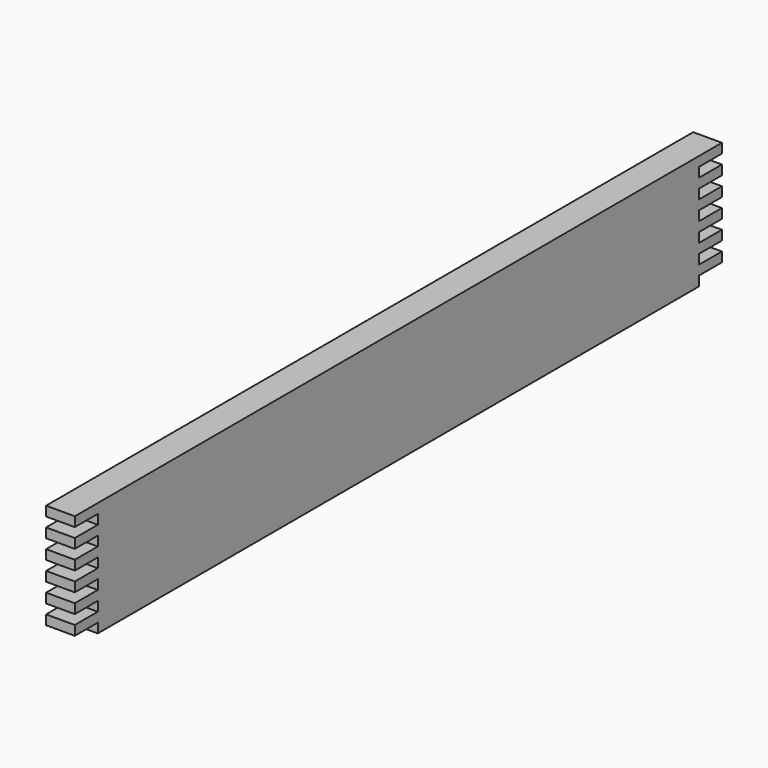
from build123d import *

# Parameters (mm, degrees)
F0_W     = 19.05
F0_H     = 76.2
F1_DEPTH = 268.351
F2_W     = 19.05
F2_H     = 6.35
F3_DEPTH = 19.051


# Not quite as in the source:
# - a pattern or mirror of a feature is missing from the dataset's text; its kind, count and spacing are read off the source's solid


with BuildPart() as f1:
    # F0 (on Front) → F1 (new body, symmetric)
    with BuildSketch(Plane.XZ):
        Rectangle(F0_W, F0_H)
    extrude(amount=F1_DEPTH, both=True)

    # F2 (on face) → F3 (cut, through all)
    with BuildSketch(Plane.YZ.offset(9.525)):
        with Locations((-258.826, 28.575)):
            Rectangle(F2_W, F2_H)
        with Locations((-258.826, 3.175)):
            Rectangle(F2_W, F2_H)
        with Locations((-258.826, -9.525)):
            Rectangle(F2_W, F2_H)
        with Locations((-258.826, -22.225)):
            Rectangle(F2_W, F2_H)
        with Locations((-258.826, 15.875)):
            Rectangle(F2_W, F2_H)
        with Locations((-258.826, -34.925)):
            Rectangle(F2_W, F2_H)
    f3 = extrude(amount=-F3_DEPTH, mode=Mode.SUBTRACT)

    # F3_copies: F3 across plane
    add(f3.mirror(Plane.ZX), mode=Mode.SUBTRACT)


solid = f1.part
